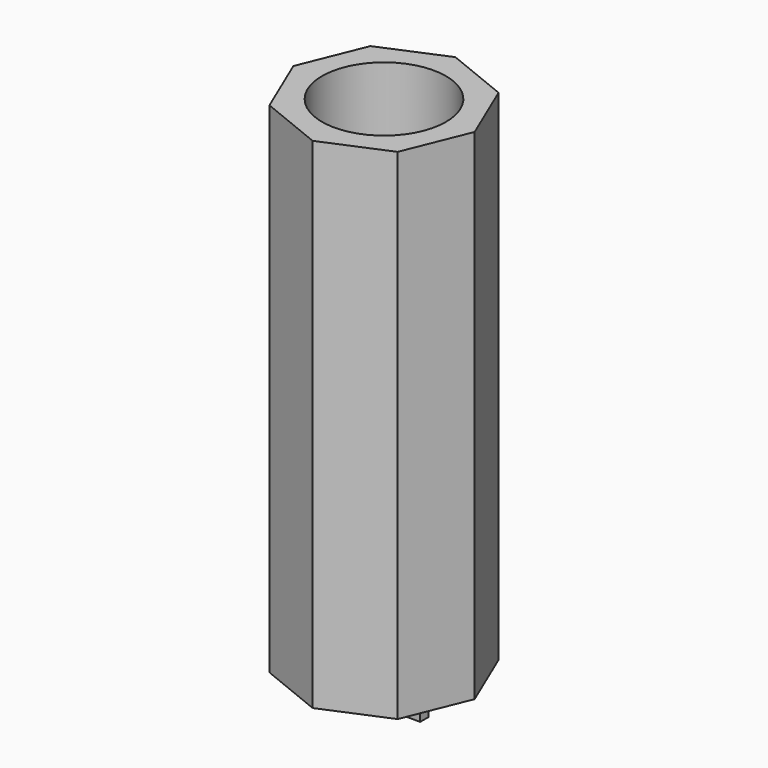
from build123d import *

# Parameters (mm, degrees)
F1_DEPTH     = 30
F2_R         = 3.725
F3_DEPTH     = 20
F4_TEXT_SIZE = 4.8611111111
F5_DEPTH     = 1


# Not quite as in the source:
# - Text() gives the source's letters only with a copy of the font that has no kerning and outlines rounded to 1/6400 em; it was checked with that copy


with BuildPart() as f1:
    # F0 (on Top) → F1 (new body)
    with BuildSketch(Plane.XY):
        Polygon((-0.0409013379, 5.4118064417), (-3.8556466467, 3.79780342), (-5.4118064417, -0.0409013379), (-3.79780342, -3.8556466467), (0.0409013379, -5.4118064417), (3.8556466467, -3.79780342), (5.4118064417, 0.0409013379), (3.79780342, 3.8556466467), align=None)
    extrude(amount=F1_DEPTH)

    # F2 (on face) → F3 (cut)
    with BuildSketch(Plane.XY.offset(30)):
        Circle(F2_R)
    extrude(amount=-F3_DEPTH, mode=Mode.SUBTRACT)

    # F4 (on face) → F5 (join)
    with BuildSketch(Plane(origin=(0, 0, 0), x_dir=(1, 0, 0), z_dir=(0, 0, -1))):
        with Locations((-3.917287838, -1.6110784908)):
            Text('D T', F4_TEXT_SIZE, font='Open Sans', font_style=FontStyle.BOLD, text_align=(TextAlign.LEFT, TextAlign.BOTTOM))
    extrude(amount=F5_DEPTH)


solid = f1.part
